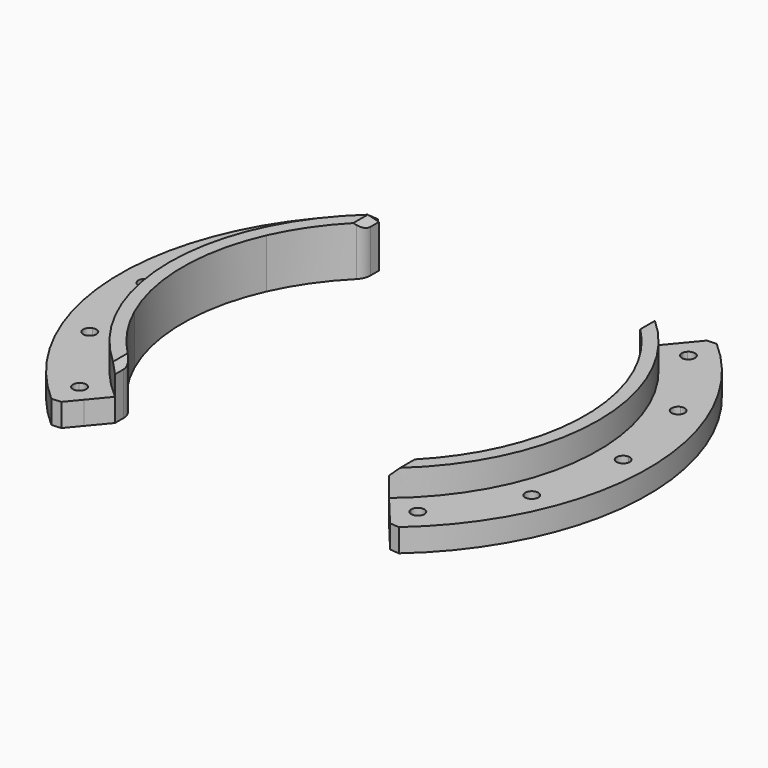
from build123d import *

# Parameters (mm, degrees)
F1_DEPTH    = 15
F2_DEPTH    = 7
F3_T1_DEPTH = 15.6101161445
F3_T3_DEPTH = 15.6101161445
F3_T5_DEPTH = 17.5438904605
F4_R        = 5


# Not quite as in the source:
# - a fillet or chamfer that OpenCascade refuses, or shapes differently, is made with other operations: its cross-section is extruded or revolved along the edge and cut away or added


with BuildPart() as f1:
    # F0 (on Top) → F1 (new body)
    with BuildSketch(Plane.XY):
        with BuildLine():
            ThreePointArc((-55.641710973, -25), (-61, 0), (-55.641710973, 25))
            ThreePointArc((-55.641710973, 25), (-49.5734728737, 35.5453342541), (-41.5331193146, 44.6766158074))
            Line((-41.5331193146, 44.6766158074), (-41.5331193146, 50))
            ThreePointArc((-41.5331193146, 50), (-65, 0), (-41.5331193146, -50))
            Line((-41.5331193146, -50), (-41.5331193146, -44.6766158074))
            ThreePointArc((-41.5331193146, -44.6766158074), (-49.5734728737, -35.5453342541), (-55.641710973, -25))
        make_face()
    extrude(amount=F1_DEPTH)

    # F0 (on Top) → F2 (join)
    with BuildSketch(Plane.XY):
        with BuildLine():
            ThreePointArc((-41.5331193146, -50), (-65, 0), (-41.5331193146, 50))
            Line((-41.5331193146, 50), (-46.3254023124, 55.7692307692))
            ThreePointArc((-46.3254023124, 55.7692307692), (-48.1036598795, 54.2428604168), (-49.8316562129, 52.6598142712))
            ThreePointArc((-49.8316562129, 52.6598142712), (-49.4122479979, 52.0178468293), (-49.265241636, 51.265241636))
            ThreePointArc((-49.265241636, 51.265241636), (-50.4871495047, 49.4228050333), (-52.6598142712, 49.8316562129))
            ThreePointArc((-52.6598142712, 49.8316562129), (-60.2815468919, 40.2788418939), (-66.1904857193, 29.581575351))
            ThreePointArc((-66.1904857193, 29.581575351), (-65.3107032116, 28.8441940675), (-64.9812661071, 27.7445488465))
            ThreePointArc((-64.9812661071, 27.7445488465), (-65.8586832477, 26.0893123909), (-67.721073831, 25.8864087733))
            ThreePointArc((-67.721073831, 25.8864087733), (-71.1069328292, 14.1440483462), (-72.4724137931, 1.9998097412))
            ThreePointArc((-72.4724137931, 1.9998097412), (-71.0760666424, 1.4044264997), (-70.5, 0))
            ThreePointArc((-70.5, 0), (-71.0760666424, -1.4044264997), (-72.4724137931, -1.9998097412))
            ThreePointArc((-72.4724137931, -1.9998097412), (-71.1069328292, -14.1440483462), (-67.721073831, -25.8864087733))
            ThreePointArc((-67.721073831, -25.8864087733), (-65.8586832477, -26.0893123909), (-64.9812661071, -27.7445488465))
            ThreePointArc((-64.9812661071, -27.7445488465), (-65.3107032116, -28.8441940675), (-66.1904857193, -29.581575351))
            ThreePointArc((-66.1904857193, -29.581575351), (-60.2815468919, -40.2788418939), (-52.6598142712, -49.8316562129))
            ThreePointArc((-52.6598142712, -49.8316562129), (-50.4871495047, -49.4228050333), (-49.265241636, -51.265241636))
            ThreePointArc((-49.265241636, -51.265241636), (-49.4122479979, -52.0178468293), (-49.8316562129, -52.6598142712))
            ThreePointArc((-49.8316562129, -52.6598142712), (-48.1036598795, -54.2428604168), (-46.3254023124, -55.7692307692))
            Line((-46.3254023124, -55.7692307692), (-41.5331193146, -50))
        make_face()
        with BuildLine():
            ThreePointArc((-49.8316562129, 52.6598142712), (-48.1036598795, 54.2428604168), (-46.3254023124, 55.7692307692))
            Line((-46.3254023124, 55.7692307692), (-51.1176853103, 61.5384615385))
            ThreePointArc((-51.1176853103, 61.5384615385), (-80, 0), (-51.1176853103, -61.5384615385))
            Line((-51.1176853103, -61.5384615385), (-46.3254023124, -55.7692307692))
            ThreePointArc((-46.3254023124, -55.7692307692), (-48.1036598795, -54.2428604168), (-49.8316562129, -52.6598142712))
            ThreePointArc((-49.8316562129, -52.6598142712), (-52.6794551984, -52.6794551984), (-52.6598142712, -49.8316562129))
            ThreePointArc((-52.6598142712, -49.8316562129), (-60.2815468919, -40.2788418939), (-66.1904857193, -29.581575351))
            ThreePointArc((-66.1904857193, -29.581575351), (-68.8290251721, -28.5099157112), (-67.721073831, -25.8864087733))
            ThreePointArc((-67.721073831, -25.8864087733), (-71.1069328292, -14.1440483462), (-72.4724137931, -1.9998097412))
            ThreePointArc((-72.4724137931, -1.9998097412), (-74.5, 0), (-72.4724137931, 1.9998097412))
            ThreePointArc((-72.4724137931, 1.9998097412), (-71.1069328292, 14.1440483462), (-67.721073831, 25.8864087733))
            ThreePointArc((-67.721073831, 25.8864087733), (-68.8290251721, 28.5099157112), (-66.1904857193, 29.581575351))
            ThreePointArc((-66.1904857193, 29.581575351), (-60.2815468919, 40.2788418939), (-52.6598142712, 49.8316562129))
            ThreePointArc((-52.6598142712, 49.8316562129), (-52.6794551984, 52.6794551984), (-49.8316562129, 52.6598142712))
        make_face()
    extrude(amount=F2_DEPTH)

    # F3: chamfer of 2 on 4 edges, made by hand

    # F3_s2 → F3_t1 (cut)
    with BuildSketch(Plane.XZ.offset(39.5332498314)):
        Polygon((-41.5331193146, 13), (-43.5331193146, 15), (-41.5331193146, 15), align=None)
    extrude(amount=F3_T1_DEPTH, mode=Mode.SUBTRACT)

    # F3_s4 → F3_t3 (cut)
    with BuildSketch(Plane.XZ.offset(-55.1433659759)):
        Polygon((-43.5331193146, 15), (-41.5331193146, 13), (-41.5331193146, 15), align=None)
    extrude(amount=F3_T3_DEPTH, mode=Mode.SUBTRACT)

    # F3_s6 → F3_t5 (cut)
    with BuildSketch(Plane.XY.offset(-5.2719452303)):
        with BuildLine():
            Line((-49.8233566102, 59.9802728911), (-52.6787878448, 60.2075187265))
            ThreePointArc((-52.6787878448, 60.2075187265), (-51.9240174848, 60.8596451538), (-51.1176853103, 61.5384615385))
            Line((-51.1176853103, 61.5384615385), (-49.8233566102, 59.9802728911))
        make_face()
        with BuildLine():
            Line((-49.8233566102, -59.9802728911), (-52.6787878448, -60.2075187265))
            ThreePointArc((-52.6787878448, -60.2075187265), (-51.9240174848, -60.8596451538), (-51.1176853103, -61.5384615385))
            Line((-51.1176853103, -61.5384615385), (-49.8233566102, -59.9802728911))
        make_face()
    extrude(amount=F3_T5_DEPTH, mode=Mode.SUBTRACT)

    # F4
    f4_edges = [f1.edges().sort_by_distance(p)[0] for p in [
        (-41.533119, 44.676616, 6.5),
        (-41.533119, -44.676616, 6.5),
    ]]
    fillet(f4_edges, radius=F4_R)


with BuildPart() as f5_1:
    # F5: instance of F1
    add(f1.part.mirror(Plane.YZ))


solid = Compound([f1.part, f5_1.part])
